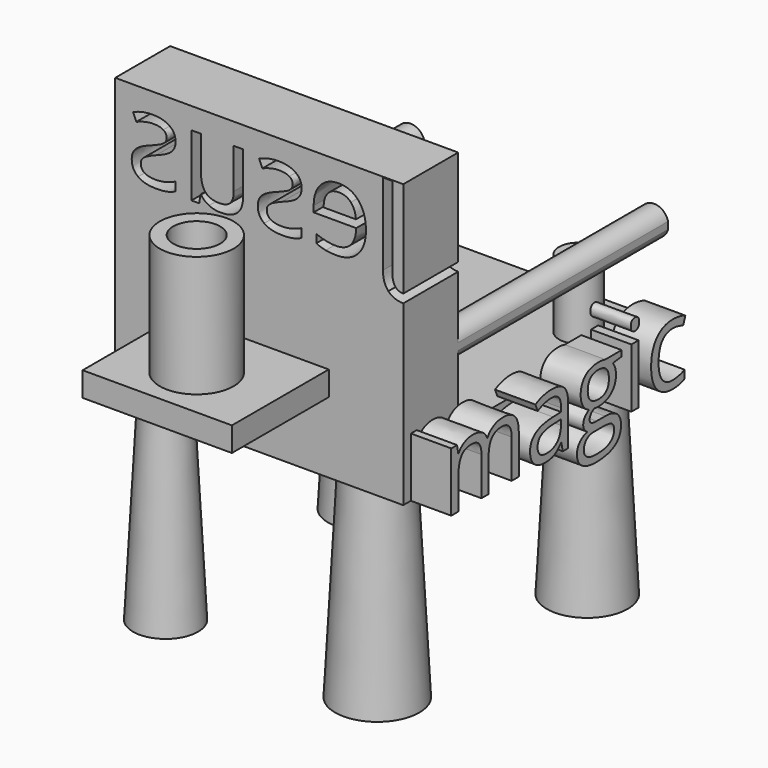
from build123d import *

# Parameters (mm, degrees)
F0_W          = 90.6265974045
F0_H          = 97.3294749856
F1_DEPTH      = 12.7
F2_R          = 8.2179047167
F3_DEPTH      = 63.5
F3_TAPER      = -3
F4_R          = 9.4116550556
F5_DEPTH      = 63.5
F5_TAPER      = -3
F6_R          = 6.9074034691
F7_DEPTH      = 63.5
F7_TAPER      = -3
F8_R          = 9.9040173916
F9_DEPTH      = 63.5
F9_TAPER      = -3
F10_W         = 90.6265974045
F10_H         = 21.6088648885
F11_DEPTH     = 76.2
F13_DEPTH     = 82.55
F14_R         = 4.4983083632
F15_DEPTH     = 82.55
F17_DEPTH     = 28.2847862691
F19_TEXT_SIZE = 19.0047547221
F20_DEPTH     = 25.4
F21_TEXT_SIZE = 16.2889197883
F22_DEPTH     = 25.4
F23_TEXT_SIZE = 14.8012820217
F24_DEPTH     = 25.4
F25_TEXT_SIZE = 19.2688389992
F26_DEPTH     = 25.4
F27_TEXT_SIZE = 34.8266040427
F28_DEPTH     = 12.7
F29_TEXT_SIZE = 17.6388888889
F30_DEPTH     = 12.7
F31_R         = 4.9826303578
F32_DEPTH     = 21.59
F33_R         = 6.1929872961
F34_DEPTH     = 21.59
F35_W         = 46.9636172056
F35_H         = 7.661037147
F36_DEPTH     = 38.1
F37_R         = 11.6201186381
F38_DEPTH     = 38.1
F39_R         = 7.3787820268
F40_DEPTH     = 25.4


# Not quite as in the source:
# - Text() gives the source's letters only with a copy of the font that has no kerning and outlines rounded to 1/6400 em; it was checked with that copy


with BuildPart() as f1:
    # F0 (on Top) → F1 (new body)
    with BuildSketch(Plane.XY):
        with Locations((-1.7846748233, 12.7436779439)):
            Rectangle(F0_W, F0_H)
    extrude(amount=F1_DEPTH)

    # F2 (on face) → F3 (join)
    with BuildSketch(Plane(origin=(0, 0, 0), x_dir=(1, 0, 0), z_dir=(0, 0, -1))):
        with Locations((-38.8800688088, -51.8569871783)):
            Circle(F2_R)
    extrude(amount=F3_DEPTH, taper=F3_TAPER)

    # F4 (on face) → F5 (join)
    with BuildSketch(Plane(origin=(0, 0, 0), x_dir=(1, 0, 0), z_dir=(0, 0, -1))):
        with Locations((32.1384854615, -50.6645701826)):
            Circle(F4_R)
    extrude(amount=F5_DEPTH, taper=F5_TAPER)

    # F8 (on face) → F9 (join)
    with BuildSketch(Plane(origin=(0, 0, 0), x_dir=(1, 0, 0), z_dir=(0, 0, -1))):
        with Locations((26.111215353, 24.3818536401)):
            Circle(F8_R)
    extrude(amount=F9_DEPTH, taper=F9_TAPER)

    # F10 (on face) → F11 (join)
    with BuildSketch(Plane.XY.offset(12.7)):
        with Locations((-1.7846748233, -25.1166271046)):
            Rectangle(F10_W, F10_H)
    extrude(amount=F11_DEPTH)

    # F12 (on face) → F13 (join)
    with BuildSketch(Plane(origin=(0, -14.3121946603, 0), x_dir=(-1, 0, 0), z_dir=(0, 1, 0))):
        with BuildLine():
            ThreePointArc((-43.528623879, 34.0761796471), (-38.5675096295, 30.6601768191), (-34.5749621454, 35.1703092456))
            ThreePointArc((-34.5749621454, 35.1703092456), (-38.5675096295, 39.680441672), (-43.528623879, 36.264438844))
            Line((-43.528623879, 36.264438844), (-43.528623879, 34.0761796471))
        make_face()
    extrude(amount=F13_DEPTH)

    # F14 (on face) → F15 (join)
    with BuildSketch(Plane(origin=(0, -14.3121946603, 0), x_dir=(-1, 0, 0), z_dir=(0, 1, 0))):
        with Locations((37.5010818243, 32.4903689325)):
            Circle(F14_R)
    extrude(amount=F15_DEPTH)

    # F16 (on face) → F17 (cut)
    with BuildSketch(Plane(origin=(0, -14.3121946603, 0), x_dir=(-1, 0, 0), z_dir=(0, 1, 0))):
        with BuildLine():
            Line((9.8135494978, 69.5591310459), (9.8135494978, 82.1803970712))
            Line((9.8135494978, 82.1803970712), (6.8314771921, 82.1803970712))
            Line((6.8314771921, 82.1803970712), (6.8314771921, 69.4512084291))
            add(Edge.make_bspline(
                [(8.5951599557, 64.0550775903), (6.8314771921, 65.7420784946), (6.8314771921, 69.4512084291)],
                knots=[0, 0, 0, 1, 1, 1], degree=2))
            add(Edge.make_bspline(
                [(13.9089287976, 62.3680766859), (10.3588427194, 62.3680766859), (8.5951599557, 64.0550775903)],
                knots=[0, 0, 0, 1, 1, 1], degree=2))
            add(Edge.make_bspline(
                [(17.578297768, 63.1320552099), (15.9708187918, 62.3680766859), (13.9089287976, 62.3680766859)],
                knots=[0, 0, 0, 1, 1, 1], degree=2))
            add(Edge.make_bspline(
                [(20.0889186425, 65.3331085784), (19.1857767442, 63.896033734), (17.578297768, 63.1320552099)],
                knots=[0, 0, 0, 1, 1, 1], degree=2))
            Line((20.0889186425, 65.3331085784), (20.2479624988, 65.3331085784))
            Line((20.2479624988, 65.3331085784), (20.6739728282, 62.7259253626))
            Line((20.6739728282, 62.7259253626), (23.1050717746, 62.7259253626))
            Line((23.1050717746, 62.7259253626), (23.1050717746, 82.1803970712))
            Line((23.1050717746, 82.1803970712), (20.1570802952, 82.1803970712))
            Line((20.1570802952, 82.1803970712), (20.1570802952, 71.9561491659))
            add(Edge.make_bspline(
                [(18.7484061394, 66.5060570187), (20.1570802952, 68.173177441), (20.1570802952, 71.9561491659)],
                knots=[0, 0, 0, 1, 1, 1], degree=2))
            add(Edge.make_bspline(
                [(14.2838178874, 64.8389365963), (17.3397319836, 64.8389365963), (18.7484061394, 66.5060570187)],
                knots=[0, 0, 0, 1, 1, 1], degree=2))
            add(Edge.make_bspline(
                [(10.8956157344, 66.0090449677), (11.977681971, 64.8389365963), (14.2838178874, 64.8389365963)],
                knots=[0, 0, 0, 1, 1, 1], degree=2))
            add(Edge.make_bspline(
                [(9.8135494978, 69.5591310459), (9.8135494978, 67.1791533391), (10.8956157344, 66.0090449677)],
                knots=[0, 0, 0, 1, 1, 1], degree=2))
        make_face()
        with BuildLine():
            add(Edge.make_bspline(
                [(2.2476060479, 68.0311739979), (2.2476060479, 65.3160681653), (0.2254770177, 63.8420724256)],
                knots=[0, 0, 0, 1, 1, 1], degree=2))
            add(Edge.make_bspline(
                [(1.0320565747, 71.2461319503), (2.2476060479, 69.9681009621), (2.2476060479, 68.0311739979)],
                knots=[0, 0, 0, 1, 1, 1], degree=2))
            add(Edge.make_bspline(
                [(-3.6426967731, 73.7851535134), (-0.1834928985, 72.5241629384), (1.0320565747, 71.2461319503)],
                knots=[0, 0, 0, 1, 1, 1], degree=2))
            add(Edge.make_bspline(
                [(-7.0507794082, 75.2250684267), (-6.164677923, 74.7280563758), (-3.6426967731, 73.7851535134)],
                knots=[0, 0, 0, 1, 1, 1], degree=2))
            add(Edge.make_bspline(
                [(-8.3373306029, 76.2702137682), (-7.9368808933, 75.7220804777), (-7.0507794082, 75.2250684267)],
                knots=[0, 0, 0, 1, 1, 1], degree=2))
            add(Edge.make_bspline(
                [(-8.7377803125, 77.6022060647), (-8.7377803125, 76.8183470586), (-8.3373306029, 76.2702137682)],
                knots=[0, 0, 0, 1, 1, 1], degree=2))
            add(Edge.make_bspline(
                [(-7.6727544891, 79.4113299302), (-8.7377803125, 78.7552740229), (-8.7377803125, 77.6022060647)],
                knots=[0, 0, 0, 1, 1, 1], degree=2))
            add(Edge.make_bspline(
                [(-4.511757845, 80.0673858374), (-6.6077286656, 80.0673858374), (-7.6727544891, 79.4113299302)],
                knots=[0, 0, 0, 1, 1, 1], degree=2))
            add(Edge.make_bspline(
                [(0.7934907902, 78.8631966397), (-2.1317801382, 80.0673858374), (-4.511757845, 80.0673858374)],
                knots=[0, 0, 0, 1, 1, 1], degree=2))
            Line((0.7934907902, 78.8631966397), (1.8443162694, 81.2602147597))
            add(Edge.make_bspline(
                [(-4.3015927492, 82.5382457479), (-1.1604765872, 82.5382457479), (1.8443162694, 81.2602147597)],
                knots=[0, 0, 0, 1, 1, 1], degree=2))
            add(Edge.make_bspline(
                [(-9.6068413845, 81.1608123495), (-7.6699144202, 82.5382457479), (-4.3015927492, 82.5382457479)],
                knots=[0, 0, 0, 1, 1, 1], degree=2))
            add(Edge.make_bspline(
                [(-11.5437683487, 77.4034012443), (-11.5437683487, 79.7833789512), (-9.6068413845, 81.1608123495)],
                knots=[0, 0, 0, 1, 1, 1], degree=2))
            add(Edge.make_bspline(
                [(-10.9842747828, 75.11714581), (-11.5437683487, 76.0742490167), (-11.5437683487, 77.4034012443)],
                knots=[0, 0, 0, 1, 1, 1], degree=2))
            add(Edge.make_bspline(
                [(-9.2802334653, 73.4045842858), (-10.4247812169, 74.1600426033), (-10.9842747828, 75.11714581)],
                knots=[0, 0, 0, 1, 1, 1], degree=2))
            add(Edge.make_bspline(
                [(-5.420579881, 71.6380614533), (-8.1356857137, 72.6491259684), (-9.2802334653, 73.4045842858)],
                knots=[0, 0, 0, 1, 1, 1], degree=2))
            add(Edge.make_bspline(
                [(-1.5751266411, 69.7295351777), (-2.5577904676, 70.5361147346), (-5.420579881, 71.6380614533)],
                knots=[0, 0, 0, 1, 1, 1], degree=2))
            add(Edge.make_bspline(
                [(-0.5924628147, 67.7869280757), (-0.5924628147, 68.9229556207), (-1.5751266411, 69.7295351777)],
                knots=[0, 0, 0, 1, 1, 1], degree=2))
            add(Edge.make_bspline(
                [(-1.8335729076, 65.5404336054), (-0.5924628147, 66.2760114408), (-0.5924628147, 67.7869280757)],
                knots=[0, 0, 0, 1, 1, 1], degree=2))
            add(Edge.make_bspline(
                [(-5.380818917, 64.80485577), (-3.0746830006, 64.80485577), (-1.8335729076, 65.5404336054)],
                knots=[0, 0, 0, 1, 1, 1], degree=2))
            add(Edge.make_bspline(
                [(-8.479334046, 65.2109856173), (-6.8746951387, 64.80485577), (-5.380818917, 64.80485577)],
                knots=[0, 0, 0, 1, 1, 1], degree=2))
            add(Edge.make_bspline(
                [(-11.4869669715, 66.3271326803), (-10.0839729534, 65.6171154647), (-8.479334046, 65.2109856173)],
                knots=[0, 0, 0, 1, 1, 1], degree=2))
            Line((-11.4869669715, 66.3271326803), (-11.4869669715, 63.5949864345))
            add(Edge.make_bspline(
                [(-5.4546607074, 62.3680766859), (-9.3228344982, 62.3680766859), (-11.4869669715, 63.5949864345)],
                knots=[0, 0, 0, 1, 1, 1], degree=2))
            add(Edge.make_bspline(
                [(0.2254770177, 63.8420724256), (-1.7966520124, 62.3680766859), (-5.4546607074, 62.3680766859)],
                knots=[0, 0, 0, 1, 1, 1], degree=2))
        make_face()
        with BuildLine():
            Line((-43.528623879, 58.5949082577), (-43.528623879, 55.8948658363))
            add(Edge.make_bspline(
                [(-38.8425102557, 57.7472846465), (-40.4885833696, 55.9558084075), (-43.528623879, 55.8948658363)],
                knots=[0, 0, 0, 0.965981926, 0.965981926, 0.965981926], degree=2))
            add(Edge.make_bspline(
                [(-37.1384689382, 62.9758514225), (-37.1384689382, 59.6018496138), (-38.8425102557, 57.7472846465)],
                knots=[0, 0, 0, 1, 1, 1], degree=2))
            Line((-37.1384689382, 62.9758514225), (-37.1384689382, 88.6784746287))
            Line((-37.1384689382, 88.6784746287), (-40.1546220702, 88.6784746287))
            Line((-40.1546220702, 88.6784746287), (-40.1546220702, 62.7259253626))
            add(Edge.make_bspline(
                [(-41.069124244, 59.6558109222), (-40.1546220702, 60.7208367456), (-40.1546220702, 62.7259253626)],
                knots=[0, 0, 0, 1, 1, 1], degree=2))
            add(Edge.make_bspline(
                [(-43.528623879, 58.5949082577), (-41.9267254418, 58.6570517632), (-41.069124244, 59.6558109222)],
                knots=[0.0622207115, 0.0622207115, 0.0622207115, 1, 1, 1], degree=2))
        make_face()
        with BuildLine():
            add(Edge.make_bspline(
                [(-22.4780334696, 62.3680766859), (-26.789258003, 62.3680766859), (-29.2856785332, 64.9979804526)],
                knots=[0, 0, 0, 1, 1, 1], degree=2))
            add(Edge.make_bspline(
                [(-19.1153919363, 62.6634438476), (-20.507025679, 62.3680766859), (-22.4780334696, 62.3680766859)],
                knots=[0, 0, 0, 1, 1, 1], degree=2))
            add(Edge.make_bspline(
                [(-16.1617203193, 63.6290672609), (-17.7237581937, 62.9588110093), (-19.1153919363, 62.6634438476)],
                knots=[0, 0, 0, 1, 1, 1], degree=2))
            Line((-16.1617203193, 63.6290672609), (-16.1617203193, 66.2589710276))
            add(Edge.make_bspline(
                [(-22.3701108528, 64.9468592131), (-19.2289946908, 64.9468592131), (-16.1617203193, 66.2589710276)],
                knots=[0, 0, 0, 1, 1, 1], degree=2))
            add(Edge.make_bspline(
                [(-26.9937429611, 66.7219022522), (-25.3521831585, 64.9468592131), (-22.3701108528, 64.9468592131)],
                knots=[0, 0, 0, 1, 1, 1], degree=2))
            add(Edge.make_bspline(
                [(-28.7261849673, 71.9220683396), (-28.6353027637, 68.4969452913), (-26.9937429611, 66.7219022522)],
                knots=[0, 0, 0, 1, 1, 1], degree=2))
            Line((-28.7261849673, 71.9220683396), (-15.3267400737, 71.9220683396))
            Line((-15.3267400737, 71.9220683396), (-15.3267400737, 73.7851535134))
            add(Edge.make_bspline(
                [(-17.4567917206, 80.1327074213), (-15.3267400737, 77.7271690947), (-15.3267400737, 73.7851535134)],
                knots=[0, 0, 0, 1, 1, 1], degree=2))
            add(Edge.make_bspline(
                [(-23.2391719248, 82.5382457479), (-19.5868433675, 82.5382457479), (-17.4567917206, 80.1327074213)],
                knots=[0, 0, 0, 1, 1, 1], degree=2))
            add(Edge.make_bspline(
                [(-29.4646028715, 79.7691786069), (-27.1471066797, 82.5382457479), (-23.2391719248, 82.5382457479)],
                knots=[0, 0, 0, 1, 1, 1], degree=2))
            add(Edge.make_bspline(
                [(-31.7820990634, 72.2912772917), (-31.7820990634, 77.0001114658), (-29.4646028715, 79.7691786069)],
                knots=[0, 0, 0, 1, 1, 1], degree=2))
            add(Edge.make_bspline(
                [(-29.2856785332, 64.9979804526), (-31.7820990634, 67.6278842194), (-31.7820990634, 72.2912772917)],
                knots=[0, 0, 0, 1, 1, 1], degree=2))
        make_face()
        with BuildLine():
            add(Edge.make_bspline(
                [(-23.2789328889, 80.0673858374), (-25.6191496316, 80.0673858374), (-27.0136234431, 78.5422688582)],
                knots=[0, 0, 0, 1, 1, 1], degree=2))
            add(Edge.make_bspline(
                [(-19.7260067418, 78.5848698912), (-20.9671168347, 80.0673858374), (-23.2789328889, 80.0673858374)],
                knots=[0, 0, 0, 1, 1, 1], degree=2))
            add(Edge.make_bspline(
                [(-18.4848966488, 74.3190864596), (-18.4848966488, 77.1023539449), (-19.7260067418, 78.5848698912)],
                knots=[0, 0, 0, 1, 1, 1], degree=2))
            Line((-18.4848966488, 74.3190864596), (-28.6580233146, 74.3190864596))
            add(Edge.make_bspline(
                [(-27.0136234431, 78.5422688582), (-28.4080972547, 77.017151879), (-28.6580233146, 74.3190864596)],
                knots=[0, 0, 0, 1, 1, 1], degree=2))
        make_face(mode=Mode.SUBTRACT)
        with BuildLine():
            add(Edge.make_bspline(
                [(41.900647507, 68.0311739979), (41.900647507, 65.3160681653), (39.8785184769, 63.8420724256)],
                knots=[0, 0, 0, 1, 1, 1], degree=2))
            add(Edge.make_bspline(
                [(40.6850980339, 71.2461319503), (41.900647507, 69.9681009621), (41.900647507, 68.0311739979)],
                knots=[0, 0, 0, 1, 1, 1], degree=2))
            add(Edge.make_bspline(
                [(36.0103446861, 73.7851535134), (39.4695485607, 72.5241629384), (40.6850980339, 71.2461319503)],
                knots=[0, 0, 0, 1, 1, 1], degree=2))
            add(Edge.make_bspline(
                [(32.602262051, 75.2250684267), (33.4883635361, 74.7280563758), (36.0103446861, 73.7851535134)],
                knots=[0, 0, 0, 1, 1, 1], degree=2))
            add(Edge.make_bspline(
                [(31.3157108562, 76.2702137682), (31.7161605659, 75.7220804777), (32.602262051, 75.2250684267)],
                knots=[0, 0, 0, 1, 1, 1], degree=2))
            add(Edge.make_bspline(
                [(30.9152611466, 77.6022060647), (30.9152611466, 76.8183470586), (31.3157108562, 76.2702137682)],
                knots=[0, 0, 0, 1, 1, 1], degree=2))
            add(Edge.make_bspline(
                [(31.9802869701, 79.4113299302), (30.9152611466, 78.7552740229), (30.9152611466, 77.6022060647)],
                knots=[0, 0, 0, 1, 1, 1], degree=2))
            add(Edge.make_bspline(
                [(35.1412836141, 80.0673858374), (33.0453127935, 80.0673858374), (31.9802869701, 79.4113299302)],
                knots=[0, 0, 0, 1, 1, 1], degree=2))
            add(Edge.make_bspline(
                [(40.4465322494, 78.8631966397), (37.521261321, 80.0673858374), (35.1412836141, 80.0673858374)],
                knots=[0, 0, 0, 1, 1, 1], degree=2))
            Line((40.4465322494, 78.8631966397), (41.4973577285, 81.2602147597))
            add(Edge.make_bspline(
                [(35.35144871, 82.5382457479), (38.4925648719, 82.5382457479), (41.4973577285, 81.2602147597)],
                knots=[0, 0, 0, 1, 1, 1], degree=2))
            add(Edge.make_bspline(
                [(30.0462000747, 81.1608123495), (31.9831270389, 82.5382457479), (35.35144871, 82.5382457479)],
                knots=[0, 0, 0, 1, 1, 1], degree=2))
            add(Edge.make_bspline(
                [(28.1092731104, 77.4034012443), (28.1092731104, 79.7833789512), (30.0462000747, 81.1608123495)],
                knots=[0, 0, 0, 1, 1, 1], degree=2))
            add(Edge.make_bspline(
                [(28.6687666763, 75.11714581), (28.1092731104, 76.0742490167), (28.1092731104, 77.4034012443)],
                knots=[0, 0, 0, 1, 1, 1], degree=2))
            add(Edge.make_bspline(
                [(30.3728079939, 73.4045842858), (29.2282602423, 74.1600426033), (28.6687666763, 75.11714581)],
                knots=[0, 0, 0, 1, 1, 1], degree=2))
            add(Edge.make_bspline(
                [(34.2324615781, 71.6380614533), (31.5173557455, 72.6491259684), (30.3728079939, 73.4045842858)],
                knots=[0, 0, 0, 1, 1, 1], degree=2))
            add(Edge.make_bspline(
                [(38.077914818, 69.7295351777), (37.0952509916, 70.5361147346), (34.2324615781, 71.6380614533)],
                knots=[0, 0, 0, 1, 1, 1], degree=2))
            add(Edge.make_bspline(
                [(39.0605786445, 67.7869280757), (39.0605786445, 68.9229556207), (38.077914818, 69.7295351777)],
                knots=[0, 0, 0, 1, 1, 1], degree=2))
            add(Edge.make_bspline(
                [(37.8194685515, 65.5404336054), (39.0605786445, 66.2760114408), (39.0605786445, 67.7869280757)],
                knots=[0, 0, 0, 1, 1, 1], degree=2))
            add(Edge.make_bspline(
                [(34.2722225422, 64.80485577), (36.5783584586, 64.80485577), (37.8194685515, 65.5404336054)],
                knots=[0, 0, 0, 1, 1, 1], degree=2))
            add(Edge.make_bspline(
                [(31.1737074131, 65.2109856173), (32.7783463205, 64.80485577), (34.2722225422, 64.80485577)],
                knots=[0, 0, 0, 1, 1, 1], degree=2))
            add(Edge.make_bspline(
                [(28.1660744877, 66.3271326803), (29.5690685058, 65.6171154647), (31.1737074131, 65.2109856173)],
                knots=[0, 0, 0, 1, 1, 1], degree=2))
            Line((28.1660744877, 66.3271326803), (28.1660744877, 63.5949864345))
            add(Edge.make_bspline(
                [(34.1983807517, 62.3680766859), (30.3302069609, 62.3680766859), (28.1660744877, 63.5949864345)],
                knots=[0, 0, 0, 1, 1, 1], degree=2))
            add(Edge.make_bspline(
                [(39.8785184769, 63.8420724256), (37.8563894467, 62.3680766859), (34.1983807517, 62.3680766859)],
                knots=[0, 0, 0, 1, 1, 1], degree=2))
        make_face()
    extrude(amount=-F17_DEPTH, mode=Mode.SUBTRACT)

    # F19 (on face) → F20 (cut)
    with BuildSketch(Plane(origin=(0, 0, -63.5), x_dir=(1, 0, 0), z_dir=(0, 0, -1))):
        with Locations((26.4527332038, -57.2246424854)):
            Text('T', F19_TEXT_SIZE, font='Open Sans', text_align=(TextAlign.LEFT, TextAlign.BOTTOM))
    extrude(amount=-F20_DEPTH, mode=Mode.SUBTRACT)

    # F21 (on face) → F22 (cut)
    with BuildSketch(Plane(origin=(0, 0, -63.5), x_dir=(1, 0, 0), z_dir=(0, 0, -1))):
        with Locations((-43.6626151204, -57.9099394381)):
            Text('C', F21_TEXT_SIZE, font='Open Sans', text_align=(TextAlign.LEFT, TextAlign.BOTTOM))
    extrude(amount=-F22_DEPTH, mode=Mode.SUBTRACT)

    # F25 (on face) → F26 (cut)
    with BuildSketch(Plane(origin=(0, 0, -63.5), x_dir=(1, 0, 0), z_dir=(0, 0, -1))):
        with Locations((20.1709121466, 17.4475181848)):
            Text('M', F25_TEXT_SIZE, font='Open Sans', text_align=(TextAlign.LEFT, TextAlign.BOTTOM))
    extrude(amount=-F26_DEPTH, mode=Mode.SUBTRACT)

    # F27 (on face) → F28 (join)
    with BuildSketch(Plane.YZ.offset(43.528623879)):
        with Locations((-35.9210595489, 0)):
            Text('magic', F27_TEXT_SIZE, font='Open Sans', text_align=(TextAlign.LEFT, TextAlign.BOTTOM))
    extrude(amount=F28_DEPTH)

    # F29 (on face) → F30 (join)
    with BuildSketch(Plane(origin=(-47.0979735255, 0, 0), x_dir=(0, -1, 0), z_dir=(-1, 0, 0))):
        with Locations((-61.4084154367, 0)):
            Text('eye', F29_TEXT_SIZE, font='Open Sans', text_align=(TextAlign.LEFT, TextAlign.BOTTOM))
    extrude(amount=F30_DEPTH)

    # F31 (on face) → F32 (join)
    with BuildSketch(Plane.XY.offset(12.7)):
        with Locations((-36.1409783363, 54.4415526092)):
            Circle(F31_R)
    extrude(amount=F32_DEPTH)

    # F33 (on face) → F34 (join)
    with BuildSketch(Plane.XY.offset(12.7)):
        with Locations((34.9105894566, 43.835490942)):
            Circle(F33_R)
    extrude(amount=F34_DEPTH)

    # F35 (on face) → F36 (join)
    with BuildSketch(Plane.XZ.offset(35.9210595489)):
        with Locations((-3.389839083, 26.1390320957)):
            Rectangle(F35_W, F35_H)
    extrude(amount=F36_DEPTH)

    # F37 (on face) → F38 (join)
    with BuildSketch(Plane.XY.offset(29.9695506692)):
        with Locations((-4.2057773098, -57.497061789)):
            Circle(F37_R)
    extrude(amount=F38_DEPTH)

    # F39 (on face) → F40 (cut)
    with BuildSketch(Plane.XY.offset(68.0695506692)):
        with Locations((-4.2057773098, -57.497061789)):
            Circle(F39_R)
    extrude(amount=-F40_DEPTH, mode=Mode.SUBTRACT)


with BuildPart() as f7:
    # F6 (on face) → F7 (new body)
    with BuildSketch(Plane(origin=(0, 0, 0), x_dir=(1, 0, 0), z_dir=(0, 0, -1))):
        with Locations((-40.1905700564, 24.7454419732)):
            Circle(F6_R)
    extrude(amount=F7_DEPTH, taper=F7_TAPER)

    # F23 (on face) → F24 (cut)
    with BuildSketch(Plane(origin=(0, 0, -63.5), x_dir=(1, 0, 0), z_dir=(0, 0, -1))):
        with Locations((-43.0054143071, 19.1541481763)):
            Text('C', F23_TEXT_SIZE, font='Open Sans', text_align=(TextAlign.LEFT, TextAlign.BOTTOM))
    extrude(amount=-F24_DEPTH, mode=Mode.SUBTRACT)


solid = Compound([f1.part, f7.part])
